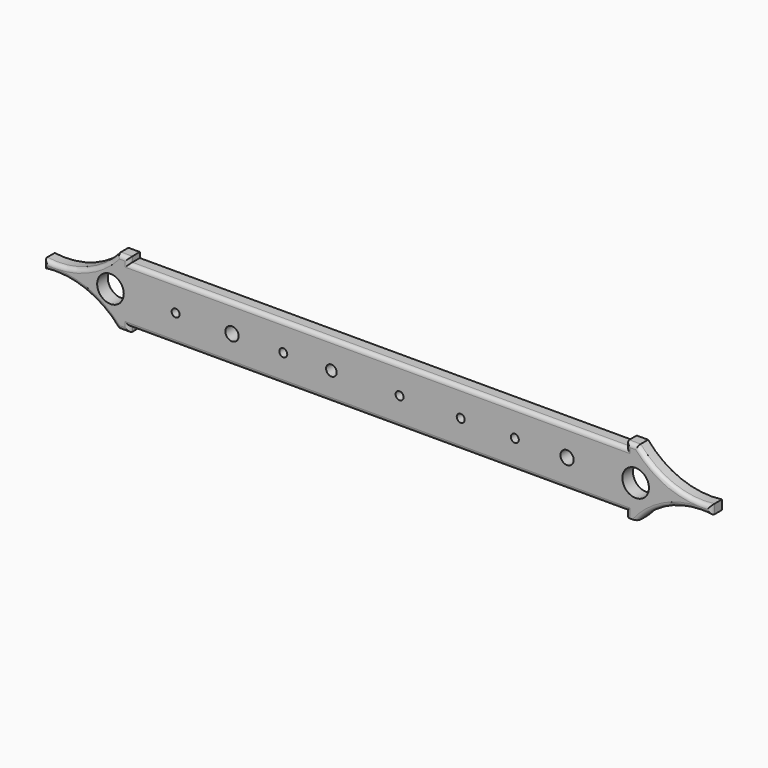
from build123d import *

# Parameters (mm, degrees)
F0_R         = 10
F0_R_2       = 3
F0_R_3       = 5
F0_R_4       = 4
F1_DEPTH     = 10
F2_T1_DEPTH  = 22
F2_T3_DEPTH  = 23.6
F2_T5_DEPTH  = 11.5
F2_T7_DEPTH  = 373.8
F2_T9_DEPTH  = 11.5
F2_T11_DEPTH = 23.6
F2_T14_ANGLE = 71.0490813257
F2_T16_ANGLE = 71.0490813257
F2_T18_ANGLE = 71.0490813257
F2_T20_ANGLE = 71.0490813257
F2_T25_DEPTH = 19
F2_T29_DEPTH = 381.3
F2_T36_DEPTH = 381.3
F2_T40_DEPTH = 19
F2_T47_DEPTH = 19
F2_T51_DEPTH = 381.3
F2_T58_DEPTH = 381.3
F2_T62_DEPTH = 19


# Not quite as in the source:
# - a fillet or chamfer that OpenCascade refuses, or shapes differently, is made with other operations: its cross-section is extruded or revolved along the edge and cut away or added


with BuildPart() as f1:
    # F0 (on Front) → F1 (new body)
    with BuildSketch(Plane.XZ):
        with BuildLine():
            ThreePointArc((251, 3.5), (220.5089399385, 7.1742403064), (195.5, 25))
            Line((195.5, 25), (186.9, 25))
            Line((186.9, 25), (186.9, 21))
            Line((186.9, 21), (-186.9, 21))
            Line((-186.9, 21), (-186.9, 25))
            Line((-186.9, 25), (-195.5, 25))
            ThreePointArc((-195.5, 25), (-220.5089399385, 7.1742403064), (-251, 3.5))
            Line((-251, 3.5), (-251, -3.5))
            ThreePointArc((-251, -3.5), (-220.5089399385, -7.1742403064), (-195.5, -25))
            Line((-195.5, -25), (-186.9, -25))
            Line((-186.9, -25), (-186.9, -21))
            Line((-186.9, -21), (186.9, -21))
            Line((186.9, -21), (186.9, -25))
            Line((186.9, -25), (195.5, -25))
            ThreePointArc((195.5, -25), (220.5089399385, -7.1742403064), (251, -3.5))
            Line((251, -3.5), (251, 3.5))
        make_face()
        with Locations((-201, 0)):
            Circle(F0_R, mode=Mode.SUBTRACT)
        with Locations((-152, 0)):
            Circle(F0_R_2, mode=Mode.SUBTRACT)
        with Locations((-109.6, 0)):
            Circle(F0_R_3, mode=Mode.SUBTRACT)
        with Locations((-71, 0)):
            Circle(F0_R_2, mode=Mode.SUBTRACT)
        with Locations((-34.8, 0)):
            Circle(F0_R_4, mode=Mode.SUBTRACT)
        with Locations((16.5, 0)):
            Circle(F0_R_2, mode=Mode.SUBTRACT)
        with Locations((62.5, 0)):
            Circle(F0_R_2, mode=Mode.SUBTRACT)
        with Locations((103.2, 0)):
            Circle(F0_R_2, mode=Mode.SUBTRACT)
        with Locations((142.5, 0)):
            Circle(F0_R_3, mode=Mode.SUBTRACT)
        with Locations((194.1, 0)):
            Circle(F0_R, mode=Mode.SUBTRACT)
    extrude(amount=F1_DEPTH)

    # F2: fillet of radius 3 on 15 edges, made by hand

    # F2_s2 → F2_t1 (cut)
    with BuildSketch(Plane.XY.offset(-11)):
        with BuildLine():
            ThreePointArc((251, -7), (250.1213203436, -9.1213203436), (248, -10))
            Line((248, -10), (251, -10))
            Line((251, -10), (251, -7))
        make_face()
        with BuildLine():
            ThreePointArc((-251, -7), (-250.1213203436, -9.1213203436), (-248, -10))
            Line((-248, -10), (-251, -10))
            Line((-251, -10), (-251, -7))
        make_face()
    extrude(amount=F2_T1_DEPTH, mode=Mode.SUBTRACT)

    # F2_s4 → F2_t3 (cut)
    with BuildSketch(Plane.YZ.offset(179.4)):
        with BuildLine():
            ThreePointArc((-7, 25), (-9.1213203436, 24.1213203436), (-10, 22))
            Line((-10, 22), (-10, 25))
            Line((-10, 25), (-7, 25))
        make_face()
    extrude(amount=F2_T3_DEPTH, mode=Mode.SUBTRACT)

    # F2_s6 → F2_t5 (cut)
    with BuildSketch(Plane.XY.offset(21)):
        with BuildLine():
            ThreePointArc((186.9, -7), (187.7786796564, -9.1213203436), (189.9, -10))
            Line((189.9, -10), (186.9, -10))
            Line((186.9, -10), (186.9, -7))
        make_face()
        with BuildLine():
            ThreePointArc((-186.9, -7), (-187.7786796564, -9.1213203436), (-189.9, -10))
            Line((-189.9, -10), (-186.9, -10))
            Line((-186.9, -10), (-186.9, -7))
        make_face()
    extrude(amount=F2_T5_DEPTH, mode=Mode.SUBTRACT)

    # F2_s8 → F2_t7 (cut)
    with BuildSketch(Plane.YZ.offset(-186.9)):
        with BuildLine():
            ThreePointArc((-7, 21), (-9.1213203436, 20.1213203436), (-10, 18))
            Line((-10, 18), (-10, 21))
            Line((-10, 21), (-7, 21))
        make_face()
        with BuildLine():
            ThreePointArc((-7, -21), (-9.1213203436, -20.1213203436), (-10, -18))
            Line((-10, -18), (-10, -21))
            Line((-10, -21), (-7, -21))
        make_face()
    extrude(amount=F2_T7_DEPTH, mode=Mode.SUBTRACT)

    # F2_s10 → F2_t9 (cut)
    with BuildSketch(Plane.XY.offset(-32.5)):
        with BuildLine():
            ThreePointArc((186.9, -7), (187.7786796564, -9.1213203436), (189.9, -10))
            Line((189.9, -10), (186.9, -10))
            Line((186.9, -10), (186.9, -7))
        make_face()
        with BuildLine():
            ThreePointArc((-186.9, -7), (-187.7786796564, -9.1213203436), (-189.9, -10))
            Line((-189.9, -10), (-186.9, -10))
            Line((-186.9, -10), (-186.9, -7))
        make_face()
    extrude(amount=F2_T9_DEPTH, mode=Mode.SUBTRACT)

    # F2_s12 → F2_t11 (cut)
    with BuildSketch(Plane.YZ.offset(-203)):
        with BuildLine():
            ThreePointArc((-7, 25), (-9.1213203436, 24.1213203436), (-10, 22))
            Line((-10, 22), (-10, 25))
            Line((-10, 25), (-7, 25))
        make_face()
        with BuildLine():
            ThreePointArc((-7, -25), (-9.1213203436, -24.1213203436), (-10, -22))
            Line((-10, -22), (-10, -25))
            Line((-10, -25), (-7, -25))
        make_face()
    extrude(amount=F2_T11_DEPTH, mode=Mode.SUBTRACT)

    # F2_s13 → F2_t14 (revolve, cut)
    with BuildSketch(Plane(origin=(243.6742780769, 0, 62.3328752784), x_dir=(0, 1, 0), z_dir=(0.9688050004, 0, 0.2478242748))):
        with BuildLine():
            ThreePointArc((-7, -59.2652075087), (-9.1213203436, -60.1438871651), (-10, -62.2652075087))
            Line((-10, -62.2652075087), (-10, -59.2652075087))
            Line((-10, -59.2652075087), (-7, -59.2652075087))
        make_face()
    revolve(axis=Axis((242.9593619468, -10, 65.127655258), (0, 1, 0)), revolution_arc=F2_T14_ANGLE, mode=Mode.SUBTRACT)

    # F2_s15 → F2_t16 (revolve, cut)
    with BuildSketch(Plane(origin=(43.3477149421, 0, 65.9912921941), x_dir=(0, 1, 0), z_dir=(-0.5490187323, 0, -0.8358100452))):
        with BuildLine():
            ThreePointArc((-7, 176.6742001078), (-9.1213203436, 175.7955204514), (-10, 173.6742001078))
            Line((-10, 173.6742001078), (-10, 176.6742001078))
            Line((-10, 176.6742001078), (-7, 176.6742001078))
        make_face()
    revolve(axis=Axis((242.9593619468, -10, -65.127655258), (0, 1, 0)), revolution_arc=F2_T16_ANGLE, mode=Mode.SUBTRACT)

    # F2_s17 → F2_t18 (revolve, cut)
    with BuildSketch(Plane(origin=(-243.6742780769, 0, -62.3328752784), x_dir=(0, 1, 0), z_dir=(-0.9688050004, 0, -0.2478242748))):
        with BuildLine():
            ThreePointArc((-7, -59.2652075087), (-9.1213203436, -60.1438871651), (-10, -62.2652075087))
            Line((-10, -62.2652075087), (-10, -59.2652075087))
            Line((-10, -59.2652075087), (-7, -59.2652075087))
        make_face()
    revolve(axis=Axis((-242.9593619468, -10, -65.127655258), (0, 1, 0)), revolution_arc=F2_T18_ANGLE, mode=Mode.SUBTRACT)

    # F2_s19 → F2_t20 (revolve, cut)
    with BuildSketch(Plane(origin=(-43.3477149421, 0, -65.9912921941), x_dir=(0, 1, 0), z_dir=(0.5490187323, 0, 0.8358100452))):
        with BuildLine():
            ThreePointArc((-7, 176.6742001078), (-9.1213203436, 175.7955204514), (-10, 173.6742001078))
            Line((-10, 173.6742001078), (-10, 176.6742001078))
            Line((-10, 176.6742001078), (-7, 176.6742001078))
        make_face()
    revolve(axis=Axis((-242.9593619468, -10, 65.127655258), (0, 1, 0)), revolution_arc=F2_T20_ANGLE, mode=Mode.SUBTRACT)


with BuildPart() as f2_tool23:
    # F2_s24 → F2_t25 (new body)
    with BuildSketch(Plane.XY.offset(32.5)):
        with BuildLine():
            ThreePointArc((186.9, -7), (187.7786796564, -9.1213203436), (189.9, -10))
            Line((189.9, -10), (186.9, -10))
            Line((186.9, -10), (186.9, -7))
        make_face()
    extrude(amount=-F2_T25_DEPTH)

    split(bisect_by=Plane.XY.offset(21), keep=Keep.BOTTOM)


with BuildPart() as f2_tool27:
    # F2_s28 → F2_t29 (new body)
    with BuildSketch(Plane.YZ.offset(194.4)):
        with BuildLine():
            ThreePointArc((-7, 21), (-9.1213203436, 20.1213203436), (-10, 18))
            Line((-10, 18), (-10, 21))
            Line((-10, 21), (-7, 21))
        make_face()
    extrude(amount=-F2_T29_DEPTH)

    split(bisect_by=Plane.YZ.offset(186.9), keep=Keep.TOP)


with BuildPart() as f2_tool23_1:
    add(f2_tool23.part)

    # F2_t31: intersect F2_tool27
    add(f2_tool27.part, mode=Mode.INTERSECT)


with BuildPart() as f1_1:
    add(f1.part)

    # F2_t21: cut F2_tool23
    add(f2_tool23_1.part, mode=Mode.SUBTRACT)


with BuildPart() as f2_tool34:
    # F2_s35 → F2_t36 (new body)
    with BuildSketch(Plane.YZ.offset(186.9)):
        with BuildLine():
            ThreePointArc((-7, 21), (-9.1213203436, 20.1213203436), (-10, 18))
            Line((-10, 18), (-10, 21))
            Line((-10, 21), (-7, 21))
        make_face()
    extrude(amount=-F2_T36_DEPTH)

    split(bisect_by=Plane.YZ.offset(-186.9), keep=Keep.BOTTOM)


with BuildPart() as f2_tool38:
    # F2_s39 → F2_t40 (new body)
    with BuildSketch(Plane.XY.offset(13.5)):
        with BuildLine():
            ThreePointArc((-186.9, -7), (-187.7786796564, -9.1213203436), (-189.9, -10))
            Line((-189.9, -10), (-186.9, -10))
            Line((-186.9, -10), (-186.9, -7))
        make_face()
    extrude(amount=F2_T40_DEPTH)

    split(bisect_by=Plane.XY.offset(21), keep=Keep.BOTTOM)


with BuildPart() as f2_tool34_1:
    add(f2_tool34.part)

    # F2_t42: intersect F2_tool38
    add(f2_tool38.part, mode=Mode.INTERSECT)


with BuildPart() as f1_2:
    add(f1_1.part)

    # F2_t32: cut F2_tool34
    add(f2_tool34_1.part, mode=Mode.SUBTRACT)


with BuildPart() as f2_tool45:
    # F2_s46 → F2_t47 (new body)
    with BuildSketch(Plane.XY.offset(-32.5)):
        with BuildLine():
            ThreePointArc((-186.9, -7), (-187.7786796564, -9.1213203436), (-189.9, -10))
            Line((-189.9, -10), (-186.9, -10))
            Line((-186.9, -10), (-186.9, -7))
        make_face()
    extrude(amount=F2_T47_DEPTH)

    split(bisect_by=Plane.XY.offset(-21), keep=Keep.TOP)


with BuildPart() as f2_tool49:
    # F2_s50 → F2_t51 (new body)
    with BuildSketch(Plane.YZ.offset(-194.4)):
        with BuildLine():
            ThreePointArc((-7, -21), (-9.1213203436, -20.1213203436), (-10, -18))
            Line((-10, -18), (-10, -21))
            Line((-10, -21), (-7, -21))
        make_face()
    extrude(amount=F2_T51_DEPTH)

    split(bisect_by=Plane.YZ.offset(-186.9), keep=Keep.BOTTOM)


with BuildPart() as f2_tool45_1:
    add(f2_tool45.part)

    # F2_t53: intersect F2_tool49
    add(f2_tool49.part, mode=Mode.INTERSECT)


with BuildPart() as f1_3:
    add(f1_2.part)

    # F2_t43: cut F2_tool45
    add(f2_tool45_1.part, mode=Mode.SUBTRACT)


with BuildPart() as f2_tool56:
    # F2_s57 → F2_t58 (new body)
    with BuildSketch(Plane.YZ.offset(-186.9)):
        with BuildLine():
            ThreePointArc((-7, -21), (-9.1213203436, -20.1213203436), (-10, -18))
            Line((-10, -18), (-10, -21))
            Line((-10, -21), (-7, -21))
        make_face()
    extrude(amount=F2_T58_DEPTH)

    split(bisect_by=Plane.YZ.offset(186.9), keep=Keep.TOP)


with BuildPart() as f2_tool60:
    # F2_s61 → F2_t62 (new body)
    with BuildSketch(Plane.XY.offset(-13.5)):
        with BuildLine():
            ThreePointArc((186.9, -7), (187.7786796564, -9.1213203436), (189.9, -10))
            Line((189.9, -10), (186.9, -10))
            Line((186.9, -10), (186.9, -7))
        make_face()
    extrude(amount=-F2_T62_DEPTH)

    split(bisect_by=Plane.XY.offset(-21), keep=Keep.TOP)


with BuildPart() as f2_tool56_1:
    add(f2_tool56.part)

    # F2_t64: intersect F2_tool60
    add(f2_tool60.part, mode=Mode.INTERSECT)


with BuildPart() as f1_4:
    add(f1_3.part)

    # F2_t54: cut F2_tool56
    add(f2_tool56_1.part, mode=Mode.SUBTRACT)


solid = f1_4.part
